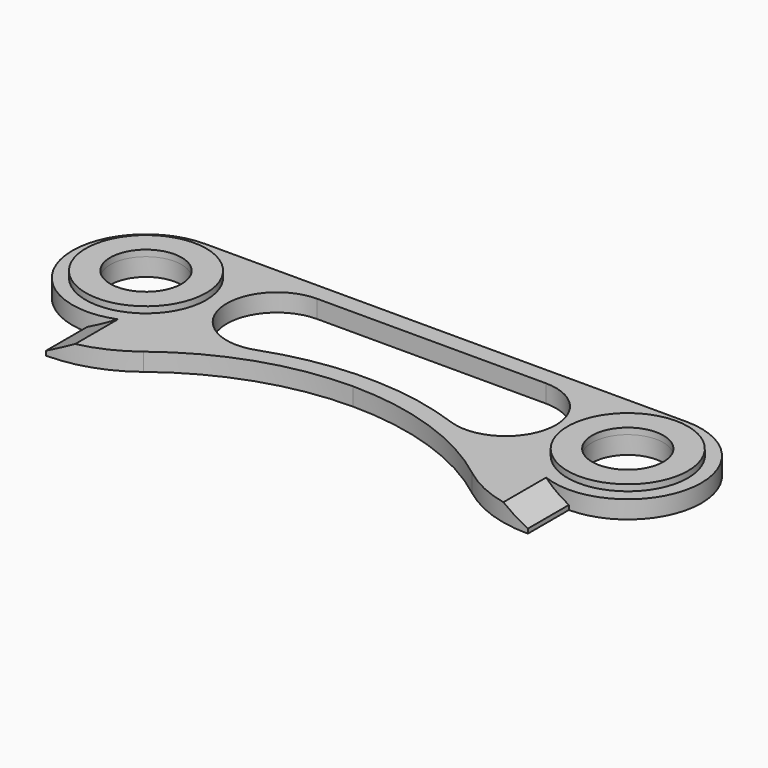
from build123d import *
from build123d import SkipClean  # not in build123d's __all__

# Parameters (mm, degrees)
F1_DEPTH = 2
F2_R     = 6.75
F2_R_2   = 4
F3_DEPTH = 0.7
F4_SIZE2 = 1.5
F4_SIZE  = 3


with BuildPart() as f1:
    # F0 (on Top) → F1 (new body)
    with BuildSketch(Plane.XY):
        with BuildLine():
            ThreePointArc((0, 8.25), (-8.25, 0), (0, -8.25))
            Line((0, -8.25), (0, -14))
            ThreePointArc((0, -14), (4.5374051759, -13.2443178107), (8.5849765979, -11.05885061))
            ThreePointArc((8.5849765979, -11.05885061), (17.2671345057, -6.3709601788), (27, -4.75))
            ThreePointArc((27, -4.75), (36.7328654943, -6.3709601788), (45.4150234021, -11.05885061))
            ThreePointArc((45.4150234021, -11.05885061), (49.4625948241, -13.2443178107), (54, -14))
            Line((54, -14), (54, -8.25))
            ThreePointArc((54, -8.25), (62.25, 0), (54, 8.25))
            Line((54, 8.25), (0, 8.25))
        make_face()
        with BuildLine():
            ThreePointArc((0, -4), (-2.8284271247, 2.8284271247), (4, 0))
            ThreePointArc((4, 0), (2.8284271247, -2.8284271247), (0, -4))
        make_face(mode=Mode.SUBTRACT)
        with BuildLine():
            Line((38.1630301369, -4.75), (38.1409883593, -4.75))
            ThreePointArc((38.1409883593, -4.75), (38.0236172708, -4.7067170267), (37.9060780323, -4.6638927855))
            ThreePointArc((37.9060780323, -4.6638927855), (27.0000000348, -2.75), (16.0939220331, -4.6638927618))
            ThreePointArc((16.0939220331, -4.6638927618), (8.6383214319, -0.3472662226), (14.1786574679, 6.25))
            Line((14.1786574679, 6.25), (39.8213425321, 6.25))
            ThreePointArc((39.8213425321, 6.25), (43.7988181762, 4.6024756442), (45.4463425321, 0.625))
            ThreePointArc((45.4463425321, 0.625), (43.1614486514, -3.9009602419), (38.1630301369, -4.75))
        make_face(mode=Mode.SUBTRACT)
        with BuildLine():
            ThreePointArc((58, 0), (56.8284271247, -2.8284271247), (54, -4))
            ThreePointArc((54, -4), (51.1715728753, 2.8284271247), (58, 0))
        make_face(mode=Mode.SUBTRACT)
    extrude(amount=F1_DEPTH)

    # F2 (on face) → F3 (join)
    with BuildSketch(Plane.XY.offset(2)):
        Circle(F2_R)
        Circle(F2_R_2, mode=Mode.SUBTRACT)
        with Locations((54, 0)):
            Circle(F2_R)
        with Locations((54, 0)):
            Circle(F2_R_2, mode=Mode.SUBTRACT)
    with SkipClean():  # cleaning this boolean's faces spoils the solid; the shape is the same uncleaned
        extrude(amount=F3_DEPTH)

    # F4
    f4_edges = [f1.edges().sort_by_distance(p)[0] for p in [
        (0, -11.125, 2),
        (54, -11.125, 2),
    ]]
    f4_side = f1.faces().sort_by_distance((49.702195, -12.544944, 2))[0]
    chamfer(f4_edges, length=F4_SIZE, length2=F4_SIZE2, reference=f4_side)


solid = f1.part
